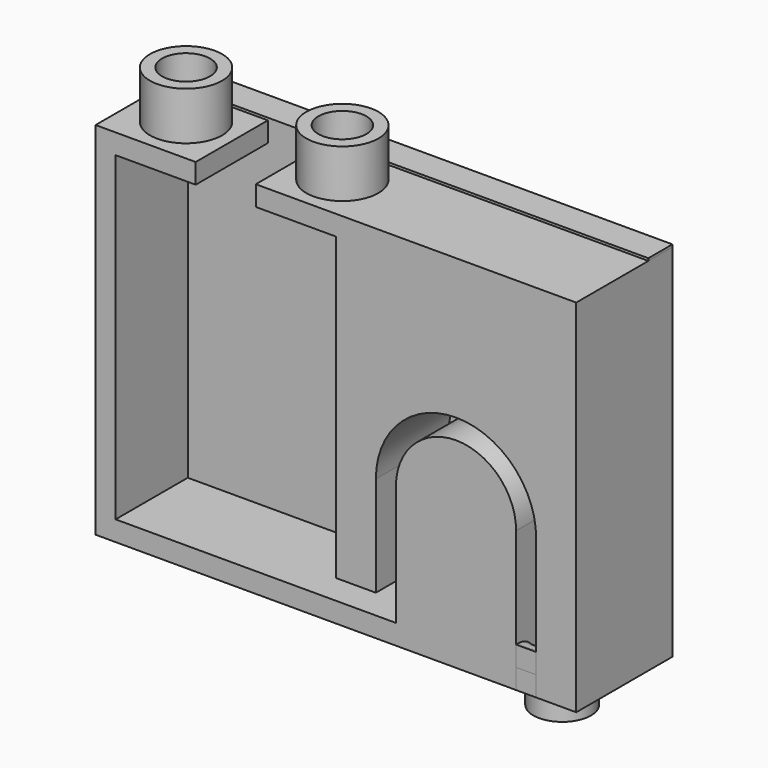
from build123d import *

# Parameters (mm, degrees)
F1_DEPTH  = 15.875
F0_W      = 2.6458333332
F0_H      = 42.3358732487
F2_W      = 63.5
F2_H      = 47.625
F2_R      = 3.175
F3_DEPTH  = 3.96875
F4_DEPTH  = 6.35
F5_R      = 4.7625
F5_R_2    = 3.175
F6_DEPTH  = 6.35
F7_R      = 3.175
F8_DEPTH  = 25.4
F9_R      = 3.81
F9_R_2    = 3.175
F10_DEPTH = 6.35
F12_DEPTH = 2.645833164
F13_DEPTH = 2.6458333316
F14_R     = 2.54
F14_2_R   = 2.54


# Not quite as in the source:
# - a feature names something its author has since deleted; it is built from what else it names


with BuildPart() as f1:
    # F0 (on Front) → F1 (new body)
    with BuildSketch(Plane.XZ):
        with BuildLine():
            Line((0, 44.979166582), (-31.75, 44.979166582))
            Line((-31.75, 44.979166582), (-31.75, 42.3358732487))
            Line((-31.75, 42.3358732487), (-31.75, 2.6458333332))
            Line((-31.75, 2.6458333332), (-26.4583333333, 2.6458333332))
            Line((-26.4583333333, 2.6458333332), (-26.4583333333, 15.875))
            ThreePointArc((-26.4583333333, 15.875), (-15.875, 26.4583333333), (-5.2916666667, 15.875))
            Line((-5.2916666667, 15.875), (-5.2916666667, 0))
            Line((-5.2916666667, 0), (0, 0))
            Line((0, 0), (0, 44.979166582))
        make_face()
        Polygon((0, -2.6458333333), (0, 0), (-5.2916666667, 0), (-5.309548229, 0), (-5.309548229, -2.6458333333), align=None)
        Polygon((-31.75, 42.3358732487), (-31.75, 44.979166582), (-34.3958333316, 44.979166582), (-37.0416664956, 44.979166582), (-42.3110765377, 44.979166582), (-42.3110765377, 42.3358732487), (-37.0416664956, 42.3358732487), (-34.3958333316, 42.3358732487), align=None)
    extrude(amount=F1_DEPTH)


with BuildPart() as f1b:
    # F0 (on Front) → F1, piece 2 (new body)
    with BuildSketch(Plane.XZ):
        with BuildLine():
            Line((-23.8125, 0), (-7.9375, 0))
            Line((-7.9375, 0), (-7.9375, 15.875))
            ThreePointArc((-7.9375, 15.875), (-15.875, 23.8125), (-23.8125, 15.875))
            Line((-23.8125, 15.875), (-23.8125, 0))
        make_face()
        Polygon((-26.4583333333, 0), (-31.75, 0), (-60.8213265341, 0), (-63.4671598673, 0), (-63.4671598673, -2.6458333333), (-7.9375, -2.6458333333), (-7.9375, 0), (-23.8125, 0), align=None)
        with Locations((-62.1442432007, 21.1679366243)):
            Rectangle(F0_W, F0_H)
        Polygon((-50.2485765377, 42.3358732487), (-50.2485765377, 44.979166582), (-55.5296598693, 44.979166582), (-58.175493201, 44.979166582), (-63.4671598673, 44.979166582), (-63.4671598673, 42.3358732487), (-60.8213265341, 42.3358732487), (-58.175493201, 42.3358732487), (-55.5296598693, 42.3358732487), align=None)
    extrude(amount=F1_DEPTH)


with BuildPart() as f3:
    # F2 (on Front) → F3 (new body)
    with BuildSketch(Plane.XZ):
        with Locations((-31.75, 21.4839725468)):
            Rectangle(F2_W, F2_H)
        with Locations((-53.975, 7.1964725468)):
            Circle(F2_R, mode=Mode.SUBTRACT)
        with Locations((-9.525, 7.1964725468)):
            Circle(F2_R, mode=Mode.SUBTRACT)
        with Locations((-52.284011212, 35.7714725468)):
            Circle(F2_R, mode=Mode.SUBTRACT)
        with Locations((-9.525, 35.7714725468)):
            Circle(F2_R, mode=Mode.SUBTRACT)
        with Locations((-52.284011212, 35.7714725468)):
            Circle(F2_R)
        with Locations((-53.975, 7.1964725468)):
            Circle(F2_R)
        with Locations((-9.525, 7.1964725468)):
            Circle(F2_R)
        with Locations((-9.525, 35.7714725468)):
            Circle(F2_R)
    extrude(amount=F3_DEPTH)


with BuildPart() as f4:
    # F2 (on Front) → F4 (new body)
    with BuildSketch(Plane.XZ):
        with Locations((-9.525, 35.7714725468)):
            Circle(F2_R)
    extrude(amount=-F4_DEPTH)


with BuildPart() as f4b:
    # F2 (on Front) → F4, piece 2 (new body)
    with BuildSketch(Plane.XZ):
        with Locations((-52.284011212, 35.7714725468)):
            Circle(F2_R)
    extrude(amount=-F4_DEPTH)


with BuildPart() as f4c:
    # F2 (on Front) → F4, piece 3 (new body)
    with BuildSketch(Plane.XZ):
        with Locations((-9.525, 7.1964725468)):
            Circle(F2_R)
    extrude(amount=-F4_DEPTH)


with BuildPart() as f4d:
    # F2 (on Front) → F4, piece 4 (new body)
    with BuildSketch(Plane.XZ):
        with Locations((-53.975, 7.1964725468)):
            Circle(F2_R)
    extrude(amount=-F4_DEPTH)


with BuildPart() as f6:
    # F5 (on face) → F6 (new body)
    with BuildSketch(Plane.XY.offset(44.979166582)):
        with Locations((-56.5985765377, -9.525)):
            Circle(F5_R)
        with Locations((-56.5985765377, -9.525)):
            Circle(F5_R_2, mode=Mode.SUBTRACT)
    extrude(amount=F6_DEPTH)


with BuildPart() as f6b:
    # F5 (on face) → F6, piece 2 (new body)
    with BuildSketch(Plane.XY.offset(44.979166582)):
        with Locations((-35.9610765377, -9.525)):
            Circle(F5_R)
        with Locations((-35.9610765377, -9.525)):
            Circle(F5_R_2, mode=Mode.SUBTRACT)
    extrude(amount=F6_DEPTH)


with BuildPart() as f8_tool:
    # F7 (on face) → F8 (new body)
    with BuildSketch(Plane.XY.offset(44.979166582)):
        with Locations((-35.9610765377, -9.525)):
            Circle(F7_R)
        with Locations((-56.5985765377, -9.525)):
            Circle(F7_R)
    extrude(amount=-F8_DEPTH)


with BuildPart() as f1_1:
    add(f1.part)

    # F8: cut by f8_tool
    add(f8_tool.part, mode=Mode.SUBTRACT)


with BuildPart() as f1b_1:
    add(f1b.part)

    # F8: cut by f8_tool
    add(f8_tool.part, mode=Mode.SUBTRACT)


with BuildPart() as f10:
    # F9 (on Top) → F10 (new body)
    with BuildSketch(Plane.XY):
        with Locations((-6.6107190214, -9.929494001)):
            Circle(F9_R)
        with Locations((-6.6107190214, -9.929494001)):
            Circle(F9_R_2, mode=Mode.SUBTRACT)
    extrude(amount=-F10_DEPTH)


with BuildPart() as f12:
    # F11 (on Top) → F12 (new body)
    with BuildSketch(Plane.XY):
        with BuildLine():
            Line((-7.958422415, -12.8011434192), (-7.958422415, -15.8794317394))
            Line((-7.958422415, -15.8794317394), (-5.3125890833, -15.8794317394))
            Line((-5.3125890833, -15.8794317394), (-5.3125890833, -12.8238909126))
            ThreePointArc((-5.3125890833, -12.8238909126), (-6.6379906914, -13.1015487096), (-7.958422415, -12.8011434192))
        make_face()
    extrude(amount=F12_DEPTH)


with BuildPart() as f12b:
    # F11 (on Top) → F12, piece 2 (new body)
    with BuildSketch(Plane.XY):
        with BuildLine():
            Line((-7.958422415, -3.9545679465), (-7.958422415, -7.0578445827))
            ThreePointArc((-7.958422415, -7.0578445827), (-6.6379906914, -6.7574392924), (-5.3125890833, -7.0350970893))
            Line((-5.3125890833, -7.0350970893), (-5.3125890833, -3.9545679465))
            Line((-5.3125890833, -3.9545679465), (-7.958422415, -3.9545679465))
        make_face()
    extrude(amount=F12_DEPTH)


with BuildPart() as f13:
    # F13 (new): a face of the model
    f13_faces = [f12.part.faces().sort_by_distance(p)[0] for p in [
        (-6.6371842751, -14.4419575778, 0),
    ]]
    extrude(f13_faces, amount=F13_DEPTH)


with BuildPart() as f13b:
    # F13#2 (new): a face of the model
    f13_2_faces = [f12b.part.faces().sort_by_distance(p)[0] for p in [
        (-6.6371697987, -5.4045252139, 0),
    ]]
    extrude(f13_2_faces, amount=F13_DEPTH)


with BuildPart() as f12b_1:
    add(f12b.part)

    # F14
    f14_edges = [f12b_1.edges().sort_by_distance(p)[0] for p in [
        (-6.637991, -6.757439, 2.645833),
    ]]
    fillet(f14_edges, radius=F14_R)


with BuildPart() as f12_1:
    add(f12.part)

    # F14#2
    f14_2_edges = [f12_1.edges().sort_by_distance(p)[0] for p in [
        (-6.637991, -13.101549, 2.645833),
    ]]
    fillet(f14_2_edges, radius=F14_2_R)


solid = Compound([f3.part, f4.part, f4b.part, f4c.part, f4d.part, f6.part, f6b.part, f1_1.part, f1b_1.part, f10.part, f13.part, f13b.part, f12b_1.part, f12_1.part])
